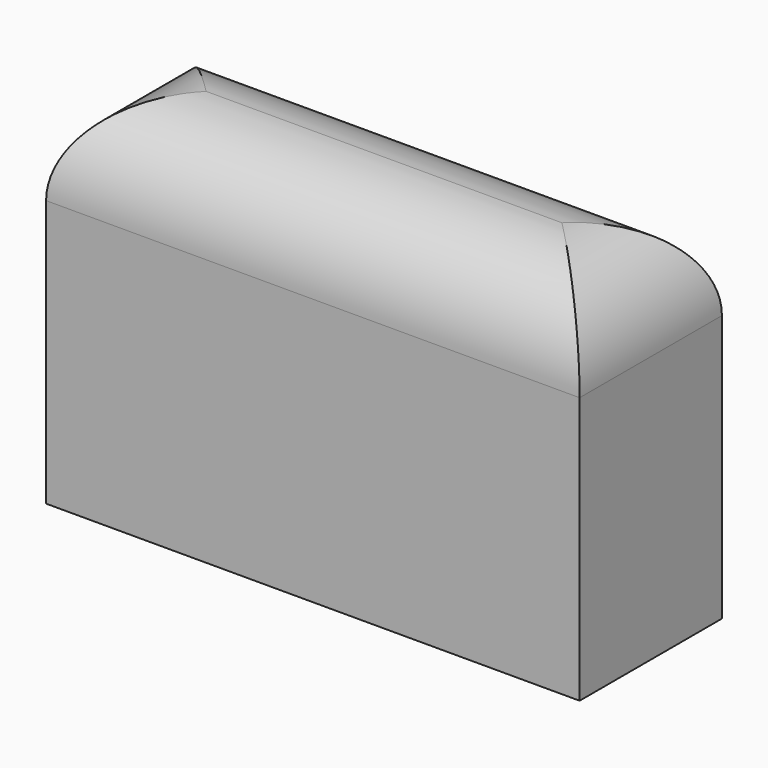
from build123d import *

# Parameters (mm, degrees)
F0_W     = 30
F0_H     = 10
F1_DEPTH = 20
F2_T     = -1.5
F3_R     = 4.99999


# Not quite as in the source:
# - a fillet or chamfer is up to 0.001 mm smaller than in the source, because OpenCascade refuses the exact size


with BuildPart() as f1:
    # F0 (on Top) → F1 (new body)
    with BuildSketch(Plane.XY):
        Rectangle(F0_W, F0_H)
    extrude(amount=F1_DEPTH)

    # F2
    f2_openings = [f1.faces().sort_by_distance(p)[0] for p in [
        (0, 0, 0),
    ]]
    offset(amount=F2_T, openings=f2_openings)

    # F3 (radius 5 in the source; OpenCascade refuses exactly that, so slightly less here)
    f3_edges = [f1.edges().sort_by_distance(p)[0] for p in [
        (-15, 0, 20),
        (0, -5, 20),
        (0, 5, 20),
        (15, 0, 20),
    ]]
    fillet(f3_edges, radius=F3_R)


solid = f1.part
